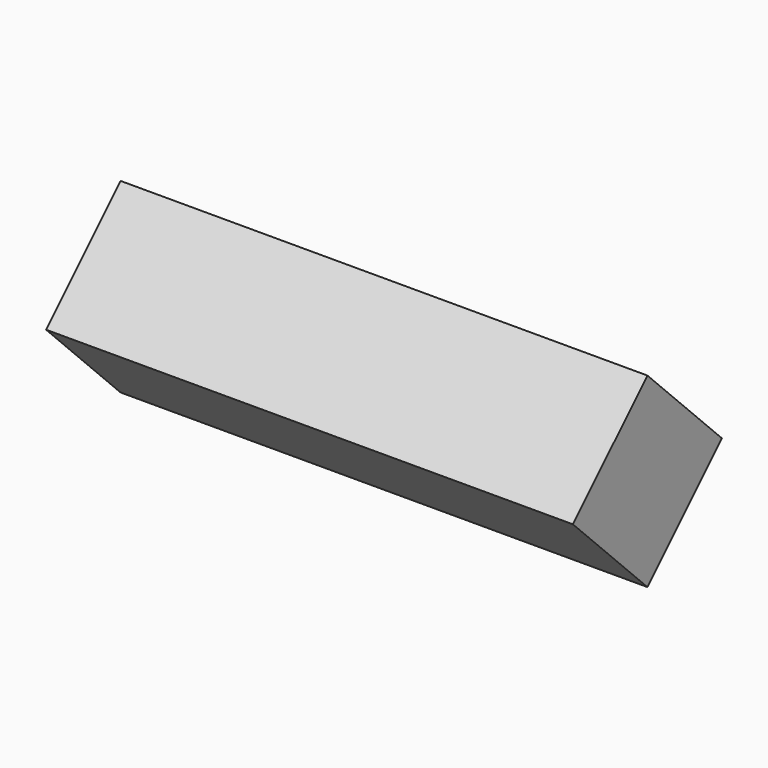
from build123d import *

# Parameters (mm, degrees)
F0_W        = 40
F0_H        = 10
F2_DEPTH    = 5
F3_ANGLE    = 45
F5_DEPTH    = 12.5
F6_T4_DEPTH = 15.1421356237
F7_T4_DEPTH = 15.1421356237


# Not quite as in the source:
# - a fillet or chamfer that OpenCascade refuses, or shapes differently, is made with other operations: its cross-section is extruded or revolved along the edge and cut away or added
# - a feature names something its author has since deleted; it is built from what else it names


with BuildPart() as f2:
    # F0 (on Top) → F2 (new body, symmetric)
    with BuildSketch(Plane.XY):
        Rectangle(F0_W, F0_H)
    extrude(amount=F2_DEPTH, both=True)


with BuildPart() as f2_1:
    # F3: moved
    add(f2.part.rotate(Axis((0, 0, 0), (-1, 0, 0)), F3_ANGLE))

    # F4 (on offset) → F5 (cut, symmetric)
    with BuildSketch(Plane.XY.offset(5)):
        Polygon((-0.8578643763, 7.0710678119), (-15, 7.0710678119), (-7.9289321881, 0), align=None)
        Polygon((15.5842712475, 7.0710678119), (1.4421356237, 7.0710678119), (8.5132034356, 0), align=None)
    extrude(amount=F5_DEPTH, both=True, mode=Mode.SUBTRACT)

    # F6: fillet of radius 0.2 on 1 edges, made by hand


with BuildPart() as f6_tool2:
    # F6_s3 → F6_t4 (new body)
    with BuildSketch(Plane.XY.offset(7.5710678119)):
        with BuildLine():
            ThreePointArc((-8.0703535444, 0.1414213562), (-7.9289321881, 0.0828427125), (-7.7875108319, 0.1414213562))
            Line((-7.7875108319, 0.1414213562), (-7.9289321881, 0))
            Line((-7.9289321881, 0), (-8.0703535444, 0.1414213562))
        make_face()
    extrude(amount=-F6_T4_DEPTH)

    split(bisect_by=Plane(origin=(0, 3.5355339059, 3.5355339059), x_dir=(1, 0, 0), z_dir=(0, -0.7071067812, -0.7071067812)), keep=Keep.TOP)

    split(bisect_by=Plane(origin=(0, 3.5355339059, -3.5355339059), x_dir=(1, 0, 0), z_dir=(0, -0.7071067812, 0.7071067812)), keep=Keep.TOP)


with BuildPart() as f2_2:
    add(f2_1.part)

    # F6_t1: union F6_tool2
    add(f6_tool2.part)

    # F7: fillet of radius 0.2 on 1 edges, made by hand


with BuildPart() as f7_tool2:
    # F7_s3 → F7_t4 (new body)
    with BuildSketch(Plane.XY.offset(7.5710678119)):
        with BuildLine():
            ThreePointArc((8.3717820794, 0.1414213562), (8.5132034356, 0.0828427125), (8.6546247918, 0.1414213562))
            Line((8.6546247918, 0.1414213562), (8.5132034356, 0))
            Line((8.5132034356, 0), (8.3717820794, 0.1414213562))
        make_face()
    extrude(amount=-F7_T4_DEPTH)

    split(bisect_by=Plane(origin=(0, 3.5355339059, -3.5355339059), x_dir=(1, 0, 0), z_dir=(0, -0.7071067812, 0.7071067812)), keep=Keep.TOP)

    split(bisect_by=Plane(origin=(0, 3.5355339059, 3.5355339059), x_dir=(1, 0, 0), z_dir=(0, -0.7071067812, -0.7071067812)), keep=Keep.TOP)


with BuildPart() as f2_3:
    add(f2_2.part)

    # F7_t1: union F7_tool2
    add(f7_tool2.part)


solid = f2_3.part
